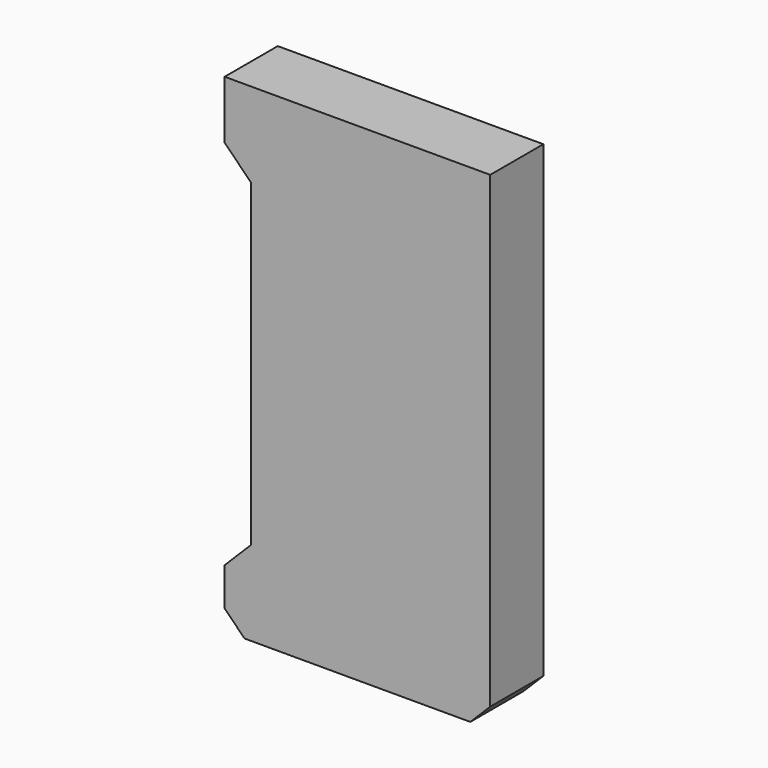
from build123d import *

# Parameters (mm, degrees)
F1_W     = 40
F1_H     = 73.52
F2_DEPTH = 10
F3_DEPTH = 4
F4_SIZE  = 3
F5_SIZE  = 3
F6_W     = 4
F6_H     = 48
F7_DEPTH = 25
F8_SIZE  = 3.99999


# Not quite as in the source:
# - a fillet or chamfer is up to 0.001 mm smaller than in the source, because OpenCascade refuses the exact size


with BuildPart() as f2:
    # F1 (on Front) → F2 (new body)
    with BuildSketch(Plane.XZ):
        Rectangle(F1_W, F1_H)
    extrude(amount=F2_DEPTH)

    # F0 (on Front) → F3 (cut)
    with BuildSketch(Plane.XZ):
        Polygon((2.3094010768, 4), (-2.3094010768, 4), (-4.6188021535, 0), (-2.3094010768, -4), (2.3094010768, -4), (4.6188021535, 0), align=None)
        Polygon((2.3094010768, 32), (-2.3094010768, 32), (-4.6188021535, 28), (-2.3094010768, 24), (2.3094010768, 24), (4.6188021535, 28), align=None)
        Polygon((2.3094010768, -24), (-2.3094010768, -24), (-4.6188021535, -28), (-2.3094010768, -32), (2.3094010768, -32), (4.6188021535, -28), align=None)
    extrude(amount=F3_DEPTH, mode=Mode.SUBTRACT)

    # F4
    f4_edges = [f2.edges().sort_by_distance(p)[0] for p in [
        (20, -5, -36.76),
    ]]
    chamfer(f4_edges, length=F4_SIZE)

    # F5
    f5_edges = [f2.edges().sort_by_distance(p)[0] for p in [
        (-20, -5, -36.76),
    ]]
    chamfer(f5_edges, length=F5_SIZE)

    # F6 (on Front) → F7 (cut)
    with BuildSketch(Plane.XZ):
        with Locations((-18, 0)):
            Rectangle(F6_W, F6_H)
    extrude(amount=F7_DEPTH, mode=Mode.SUBTRACT)

    # F8 (size 4 in the source; OpenCascade refuses exactly that, so slightly less here)
    f8_edges = [f2.edges().sort_by_distance(p)[0] for p in [
        (-20, -5, 24),
        (-20, -5, -24),
    ]]
    chamfer(f8_edges, length=F8_SIZE)


solid = f2.part
